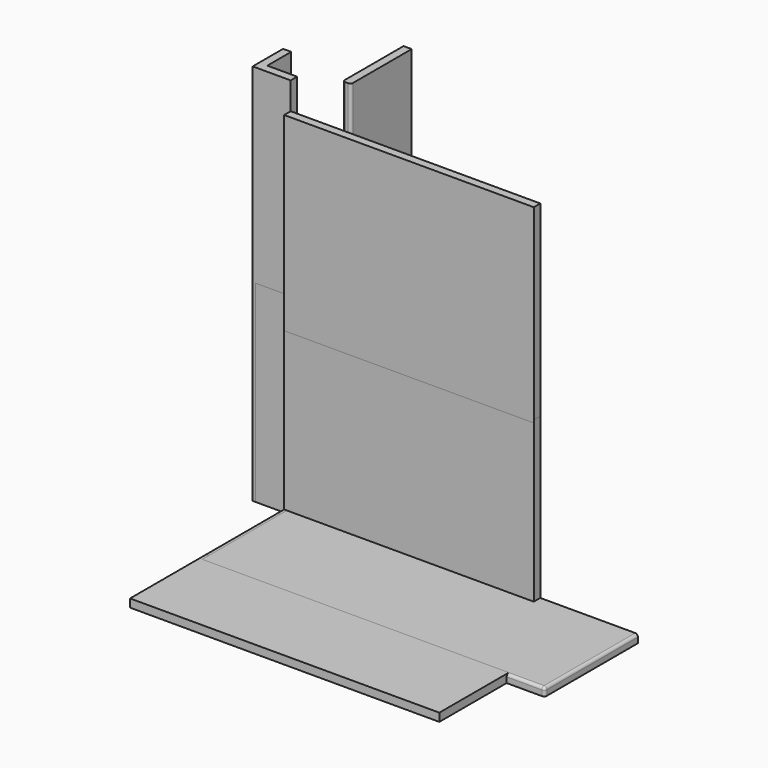
from build123d import *

# Parameters (mm, degrees)
F0_W         = 584.2
F0_H         = 19.05
F1_DEPTH     = 831.85
F2_W         = 723.9
F2_H         = 469.9
F3_DEPTH     = 19.05
F4_W         = 723.9
F4_H         = 254
F5_DEPTH     = 19.05
F6_W         = 812.8
F6_H         = 273.05
F7_DEPTH     = 19.05
F9_DEPTH     = 457.2
F11_DEPTH    = 895.35
F14_DEPTH    = 19.05
F15_DEPTH    = 19.05
F16_W        = 584.2
F16_H        = 393.7
F17_DEPTH    = 19.05
F18_R        = 6.35
F19_R        = 6.35
F20_R        = 6.35
F21_R        = 6.35
F22_R        = 6.35
F23_R        = 6.35
F24_R        = 6.35
F25_T1_DEPTH = 466.725
F25_S5_W     = 6.35
F25_S5_H     = 6.35
F25_T6_DEPTH = 6.35


# Not quite as in the source:
# - a fillet or chamfer that OpenCascade refuses, or shapes differently, is made with other operations: its cross-section is extruded or revolved along the edge and cut away or added


with BuildPart() as f1:
    # F0 (on Top) → F1 (new body)
    with BuildSketch(Plane.XY):
        with Locations((292.1, -9.525)):
            Rectangle(F0_W, F0_H)
    extrude(amount=F1_DEPTH)


with BuildPart() as f3:
    # F2 (on Top) → F3 (new body)
    with BuildSketch(Plane.XY):
        with Locations((361.95, -234.95)):
            Rectangle(F2_W, F2_H)
    extrude(amount=F3_DEPTH)


with BuildPart() as f5:
    # F4 (on Top) → F5 (new body)
    with BuildSketch(Plane.XY):
        with Locations((361.95, -127)):
            Rectangle(F4_W, F4_H)
    extrude(amount=F5_DEPTH)

    # F22
    f22_edges = [f5.edges().sort_by_distance(p)[0] for p in [
        (361.95, -254, 19.05),
        (361.95, -254, 0),
    ]]
    fillet(f22_edges, radius=F22_R)


with BuildPart() as f7:
    # F6 (on Top) → F7 (new body)
    with BuildSketch(Plane.XY):
        with Locations((406.4, -136.525)):
            Rectangle(F6_W, F6_H)
    extrude(amount=F7_DEPTH)

    # F18
    f18_edges = [f7.edges().sort_by_distance(p)[0] for p in [
        (0, -273.05, 9.525),
        (812.8, -273.05, 9.525),
        (812.8, -136.525, 19.05),
        (406.4, -273.05, 19.05),
        (0, -136.525, 19.05),
    ]]
    fillet(f18_edges, radius=F18_R)


with BuildPart() as f9:
    # F8 (on Top) → F9 (new body)
    with BuildSketch(Plane.XY):
        Polygon((-88.9, 0), (0, 0), (0, 19.05), (-69.85, 19.05), (-69.85, 88.9), (-88.9, 88.9), align=None)
    extrude(amount=F9_DEPTH)

    # F20
    f20_edges = [f9.edges().sort_by_distance(p)[0] for p in [
        (-44.45, 0, 457.2),
        (-88.9, 44.45, 457.2),
        (-69.85, 53.975, 457.2),
        (-34.925, 19.05, 457.2),
    ]]
    fillet(f20_edges, radius=F20_R)

    # F25: fillet of radius 6.35 on 2 edges, made by hand

    # F25_s2 → F25_t1 (cut)
    with BuildSketch(Plane.XY.offset(-15.875)):
        with BuildLine():
            ThreePointArc((-82.55, 0), (-87.0401280605, 1.8598719395), (-88.9, 6.35))
            Line((-88.9, 6.35), (-88.9, 0))
            Line((-88.9, 0), (-82.55, 0))
        make_face()
    extrude(amount=F25_T1_DEPTH, mode=Mode.SUBTRACT)


with BuildPart() as f11:
    # F10 (on Top) → F11 (new body)
    with BuildSketch(Plane.XY):
        Polygon((-88.9, 0), (0, 0), (0, 19.05), (-69.85, 19.05), (-69.85, 88.9), (-88.9, 88.9), (-88.9, 19.05), align=None)
    extrude(amount=F11_DEPTH)


with BuildPart() as f14:
    # F12 (on Right) → F14 (new body)
    with BuildSketch(Plane.YZ):
        Polygon((551.983873911, 795.822240965), (177.333873911, 421.172240965), (177.333873911, 295.44865527), (551.983873911, 670.09865527), align=None)
    extrude(amount=F14_DEPTH)


with BuildPart() as f15:
    # F13 (on Right) → F15 (new body)
    with BuildSketch(Plane.YZ):
        Polygon((0, 393.7), (0, 0), (330.2, 0), (330.2, 831.85), (152.4, 831.85), (152.4, 577.85), align=None)
    extrude(amount=F15_DEPTH)

    # F21
    f21_edges = [f15.edges().sort_by_distance(p)[0] for p in [
        (19.05, 76.2, 485.775),
        (0, 76.2, 485.775),
    ]]
    fillet(f21_edges, radius=F21_R)

    # F23
    f23_edges = [f15.edges().sort_by_distance(p)[0] for p in [
        (19.05, 165.1, 0),
        (0, 165.1, 0),
    ]]
    fillet(f23_edges, radius=F23_R)

    # F24
    f24_edges = [f15.edges().sort_by_distance(p)[0] for p in [
        (19.05, 152.4, 704.85),
        (0, 152.4, 704.85),
    ]]
    fillet(f24_edges, radius=F24_R)


with BuildPart() as f17:
    # F16 (on Front) → F17 (new body)
    with BuildSketch(Plane.XZ):
        with Locations((292.1, 196.85)):
            Rectangle(F16_W, F16_H)
    extrude(amount=F17_DEPTH)

    # F19
    f19_edges = [f17.edges().sort_by_distance(p)[0] for p in [
        (292.1, -19.05, 393.7),
        (292.1, 0, 393.7),
        (292.1, -19.05, 0),
    ]]
    fillet(f19_edges, radius=F19_R)


with BuildPart() as f25_tool4:
    # F25_s5 → F25_t6 (new body)
    with BuildSketch(Plane.XZ.offset(-6.35)):
        with Locations((-85.725, 454.025)):
            Rectangle(F25_S5_W, F25_S5_H)
    extrude(amount=F25_T6_DEPTH)

    # F25_s7 → F25_t8 (revolve, cut)
    with BuildSketch(Plane(origin=(-82.55, 6.35, 450.85), x_dir=(0.7071067812, 0, -0.7071067812), z_dir=(-0.7071067812, 0, -0.7071067812))):
        with BuildLine():
            ThreePointArc((0, -6.35), (6.35, 0), (0, 6.35))
            Line((0, 6.35), (0, -6.35))
        make_face()
    revolve(axis=Axis((-82.55, 6.35, 450.85), (0, -1, 0)), mode=Mode.SUBTRACT)


with BuildPart() as f9_1:
    add(f9.part)

    # F25_t3: cut F25_tool4
    add(f25_tool4.part, mode=Mode.SUBTRACT)


solid = Compound([f1.part, f3.part, f5.part, f7.part, f11.part, f15.part, f17.part, f9_1.part])
